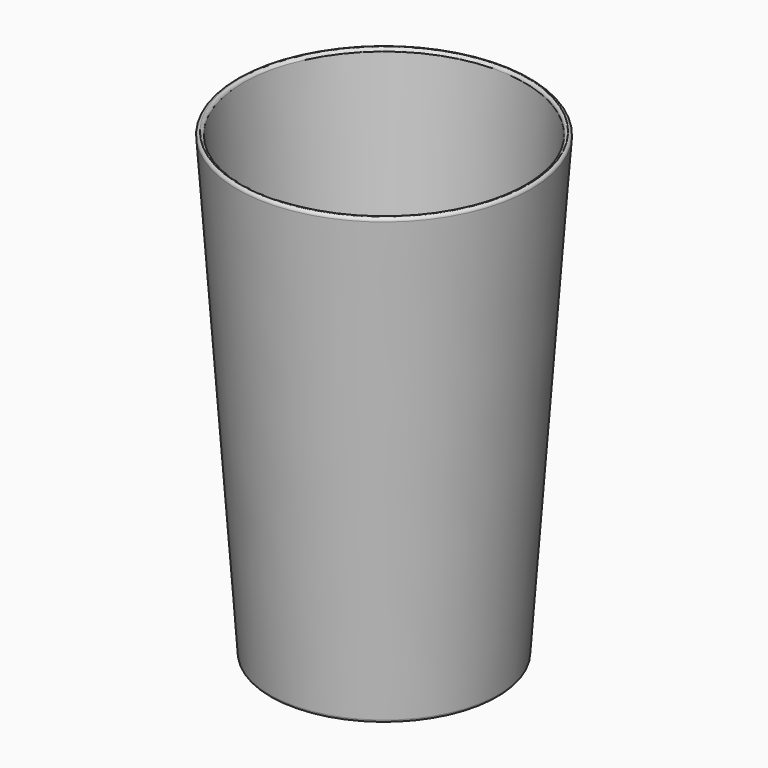
from build123d import *

# Parameters (mm, degrees)
F2_R = 0.59999


# Not quite as in the source:
# - a fillet or chamfer is up to 0.001 mm smaller than in the source, because OpenCascade refuses the exact size


with BuildPart() as f1:
    # F0 (on Front) → F1 (revolve)
    with BuildSketch(Plane.XZ):
        Polygon((-27.7969426702, 91), (-29, 91), (-22.5, 0), (0, 0), (0, 1.2), (-21.3826569559, 1.2), align=None)
    revolve(axis=Axis((0, 0, 25.3364025), (0, 0, 1)))

    # F2 (radius 0.6 in the source; OpenCascade refuses exactly that, so slightly less here)
    f2_edges = [f1.edges().sort_by_distance(p)[0] for p in [
        (27.796943, 0, 91),
        (29, 0, 91),
        (21.382657, 0, 1.2),
        (22.5, 0, 0),
    ]]
    fillet(f2_edges, radius=F2_R)


solid = f1.part
